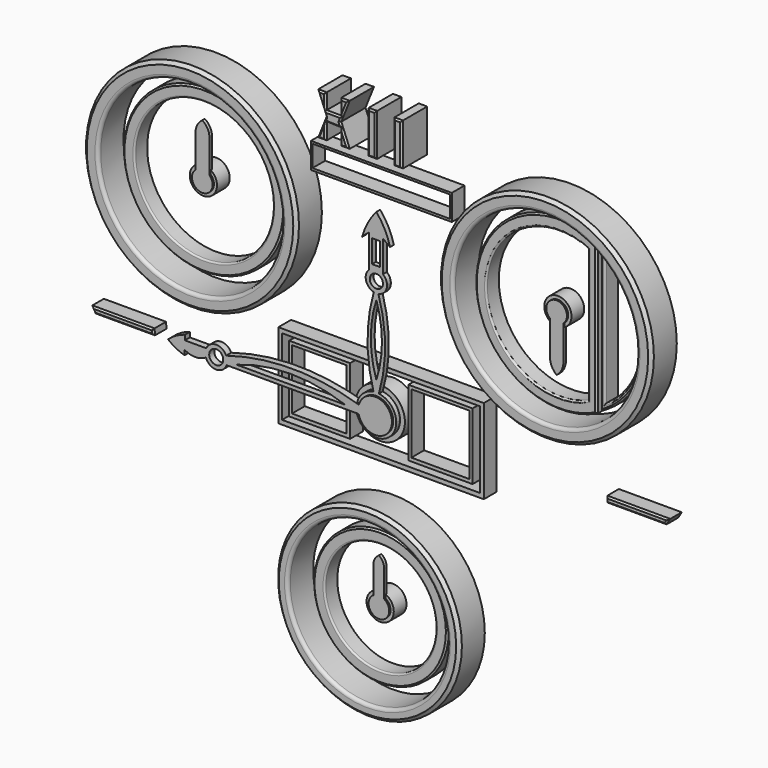
from build123d import *

# Parameters (mm, degrees)
F0_R             = 3.9514377986
F0_R_2           = 2.5863857563
F9_DEPTH         = 2.54
F1_R             = 14.6787999348
F1_R_2           = 12.7425171284
F10_DEPTH        = 5.08
F1_R_3           = 17.0073484495
F1_R_4           = 14.6752720021
F1_R_5           = 17.0023516015
F1_R_6           = 14.6892793779
F1_W             = 1.3462
F1_H             = 6.7620016634
F1_W_2           = 1.3524000533
F2_R             = 2.177276794
F2_R_2           = 1.3961214572
F11_DEPTH        = 2.54
F2_R_3           = 2.1717
F2_R_4           = 1.397
F12_DEPTH        = 2.54
F13_START        = 2.54
F13_DEPTH        = 0.762
F5_R             = 12.9377790339
F5_R_2           = 11.0821270388
F14_DEPTH        = 2.54
F5_R_3           = 10.7502912607
F5_R_4           = 8.8849316167
F15_START        = 2.54
F6_R             = 1.1208583818
F15_DEPTH        = 1.016
F7_W             = 10.2515760809
F7_H             = 10.6458668597
F7_W_2           = 9.2743812129
F7_H_2           = 9.6200094558
F16_DEPTH        = 2.54
F7_W_3           = 9.7352196462
F7_W_4           = 8.6983321235
F7_W_5           = 22.5069178268
F7_H_3           = 4.1028223932
F7_W_6           = 21.9573201612
F7_H_4           = 3.4244768322
F17_START        = 2.286
F17_DEPTH        = 0.508
F18_SIZE         = 0.508
F18_2_SIZE       = 0.508
F18_3_SIZE       = 0.508
F19_R            = 0.508
F19_2_R          = 0.508
F19_3_R          = 0.508
F20_SIZE         = 0.254
F20_2_SIZE       = 0.254
F20_3_SIZE       = 0.254
F20_4_SIZE       = 0.254
F21_R            = 0.254
F21_2_R          = 0.254
F21_3_R          = 0.254
F21_4_R          = 0.254
F22_C1_SIZE      = 0.254
F22_C2_SIZE      = 0.254
F22_C3_SIZE      = 0.254
F22_C4_SIZE      = 0.254
F22_2_C1_SIZE    = 0.254
F22_2_C2_SIZE    = 0.254
F22_2_C3_SIZE    = 0.254
F22_2_C4_SIZE    = 0.254
F22_3_T1_DEPTH   = 2.6588161753
F22_3_T3_DEPTH   = 3.1555706541
F22_3_T5_DEPTH   = 2.3183985613
F22_3_T7_DEPTH   = 2.6588164082
F22_3_T12_DEPTH  = 4.9478647113
F22_3_T17_DEPTH  = 4.9478647113
F22_3_T22_DEPTH  = 3.9716552755
F22_3_T27_DEPTH  = 3.6261524815
F22_3_T33_DEPTH  = 3.8928498877
F22_3_T38_DEPTH  = 4.9478646249
F22_3_T43_DEPTH  = 4.9478646249
F22_3_T49_DEPTH  = 3.1555706541
F22_3_T54_DEPTH  = 2.9716060403
F22_3_T62_DEPTH  = 2.9716060403
F22_3_T67_DEPTH  = 3.1555706541
F22_3_T75_DEPTH  = 4.9478647113
F22_3_T79_DEPTH  = 4.9478647113
F22_3_T86_DEPTH  = 3.3184477965
F22_3_T91_DEPTH  = 3.6261524815
F22_3_T99_DEPTH  = 3.6261524815
F22_3_T104_DEPTH = 3.2396424088
F22_3_T112_DEPTH = 4.9478646249
F22_3_T116_DEPTH = 4.9478646249
F22_4_C1_SIZE    = 0.254
F22_4_C2_SIZE    = 0.254
F22_4_C3_SIZE    = 0.254
F22_4_C4_SIZE    = 0.254
F22_5_C1_SIZE    = 0.254
F22_5_C2_SIZE    = 0.254
F22_5_C3_SIZE    = 0.254
F22_5_C4_SIZE    = 0.254


# Not quite as in the source:
# - a fillet or chamfer that OpenCascade refuses, or shapes differently, is made with other operations: its cross-section is extruded or revolved along the edge and cut away or added


with BuildPart() as f9:
    # F0 (on Front) → F9 (new body)
    with BuildSketch(Plane.XZ):
        Circle(F0_R)
        Circle(F0_R_2, mode=Mode.SUBTRACT)
    extrude(amount=F9_DEPTH)


with BuildPart() as f10:
    # F1 (on Front) → F10 (new body)
    with BuildSketch(Plane.XZ):
        with Locations((0, -27.1976441145)):
            Circle(F1_R)
        with Locations((0, -27.1976441145)):
            Circle(F1_R_2, mode=Mode.SUBTRACT)
    extrude(amount=F10_DEPTH)

    # F18
    f18_edges = [f10.edges().sort_by_distance(p)[0] for p in [
        (-14.6788, -5.08, -27.197644),
    ]]
    chamfer(f18_edges, length=F18_SIZE)

    # F19
    f19_edges = [f10.edges().sort_by_distance(p)[0] for p in [
        (-12.742517, -5.08, -27.197644),
    ]]
    fillet(f19_edges, radius=F19_R)


with BuildPart() as f10b:
    # F1 (on Front) → F10, piece 2 (new body)
    with BuildSketch(Plane.XZ):
        with Locations((-28.3488668501, 23.4561692923)):
            Circle(F1_R_3)
        with Locations((-28.3488668501, 23.4561692923)):
            Circle(F1_R_4, mode=Mode.SUBTRACT)
    extrude(amount=F10_DEPTH)

    # F18#2
    f18_2_edges = [f10b.edges().sort_by_distance(p)[0] for p in [
        (-45.356215, -5.08, 23.456169),
    ]]
    chamfer(f18_2_edges, length=F18_2_SIZE)

    # F19#2
    f19_2_edges = [f10b.edges().sort_by_distance(p)[0] for p in [
        (-43.024139, -5.08, 23.456169),
    ]]
    fillet(f19_2_edges, radius=F19_2_R)


with BuildPart() as f10c:
    # F1 (on Front) → F10, piece 3 (new body)
    with BuildSketch(Plane.XZ):
        with Locations((28.3464, 23.4561692923)):
            Circle(F1_R_5)
        with Locations((28.3464, 23.4561692923)):
            Circle(F1_R_6, mode=Mode.SUBTRACT)
    extrude(amount=F10_DEPTH)

    # F18#3
    f18_3_edges = [f10c.edges().sort_by_distance(p)[0] for p in [
        (11.344048, -5.08, 23.456169),
    ]]
    chamfer(f18_3_edges, length=F18_3_SIZE)

    # F19#3
    f19_3_edges = [f10c.edges().sort_by_distance(p)[0] for p in [
        (13.657121, -5.08, 23.456169),
    ]]
    fillet(f19_3_edges, radius=F19_3_R)


with BuildPart() as f10d:
    # F1 (on Front) → F10, piece 4 (new body)
    with BuildSketch(Plane.XZ):
        with Locations((0.6731, 40.4530894011)):
            Rectangle(F1_W, F1_H)
    extrude(amount=F10_DEPTH)

    # F22: chamfer of 0.254 on 4 edges, made by hand

    # F22_c1
    f22_c1_edges = [f10d.edges().sort_by_distance(p)[0] for p in [
        (0.6731, -5.08, 43.8340902328),
    ]]
    chamfer(f22_c1_edges, length=F22_C1_SIZE)

    # F22_c2
    f22_c2_edges = [f10d.edges().sort_by_distance(p)[0] for p in [
        (0, -5.08, 40.3260894011),
    ]]
    chamfer(f22_c2_edges, length=F22_C2_SIZE)

    # F22_c3
    f22_c3_edges = [f10d.edges().sort_by_distance(p)[0] for p in [
        (0.8001, -5.08, 37.0720885694),
    ]]
    chamfer(f22_c3_edges, length=F22_C3_SIZE)

    # F22_c4
    f22_c4_edges = [f10d.edges().sort_by_distance(p)[0] for p in [
        (1.3462, -5.08, 40.4530894011),
    ]]
    chamfer(f22_c4_edges, length=F22_C4_SIZE)


with BuildPart() as f10e:
    # F1 (on Front) → F10, piece 5 (new body)
    with BuildSketch(Plane.XZ):
        with Locations((4.7994630877, 40.4530894011)):
            Rectangle(F1_W_2, F1_H)
    extrude(amount=F10_DEPTH)

    # F22#2: chamfer of 0.254 on 4 edges, made by hand

    # F22_2_c1
    f22_2_c1_edges = [f10e.edges().sort_by_distance(p)[0] for p in [
        (4.7994630877, -5.08, 43.8340902328),
    ]]
    chamfer(f22_2_c1_edges, length=F22_2_C1_SIZE)

    # F22_2_c2
    f22_2_c2_edges = [f10e.edges().sort_by_distance(p)[0] for p in [
        (4.123263061, -5.08, 40.3260894011),
    ]]
    chamfer(f22_2_c2_edges, length=F22_2_C2_SIZE)

    # F22_2_c3
    f22_2_c3_edges = [f10e.edges().sort_by_distance(p)[0] for p in [
        (4.9264630877, -5.08, 37.0720885694),
    ]]
    chamfer(f22_2_c3_edges, length=F22_2_C3_SIZE)

    # F22_2_c4
    f22_2_c4_edges = [f10e.edges().sort_by_distance(p)[0] for p in [
        (5.4756631143, -5.08, 40.4530894011),
    ]]
    chamfer(f22_2_c4_edges, length=F22_2_C4_SIZE)


with BuildPart() as f10f:
    # F1 (on Front) → F10, piece 6 (new body)
    with BuildSketch(Plane.XZ):
        Polygon((-3.0251389835, 43.8340902328), (-4.3775402009, 43.8340902328), (-4.3775402009, 41.3317270577), (-4.3775402009, 40.4530894011), align=None)
        Polygon((-4.3775402009, 40.4530894011), (-4.3775402009, 41.3317270577), (-6.6959387623, 41.3317270577), (-6.6959387623, 40.4530894011), (-6.6959387623, 39.737328887), (-4.3775402009, 39.6585234992), align=None)
        Polygon((-3.0251389835, 37.0720885694), (-4.3775402009, 40.4530894011), (-4.3775402009, 39.6585234992), (-4.3775402009, 37.0720885694), align=None)
        Polygon((-6.6959387623, 40.4530894011), (-6.6959387623, 41.3317270577), (-6.6959387623, 43.8340902328), (-8.0483402126, 43.8340902328), align=None)
        Polygon((-6.6959387623, 39.737328887), (-6.6959387623, 40.4530894011), (-8.0483402126, 37.0720885694), (-6.6959387623, 37.0720885694), align=None)
    extrude(amount=F10_DEPTH)

    # F22#3: chamfer of 0.254 on 14 edges, made by hand

    # F22_3_s2 → F22_3_t1 (cut)
    with BuildSketch(Plane.YZ.offset(-5.0307476799)):
        Polygon((-4.826, 43.8340902328), (-5.08, 43.5800902328), (-5.08, 43.8340902328), align=None)
        Polygon((-4.826, 37.0720885694), (-5.08, 37.3260885694), (-5.08, 37.0720885694), align=None)
    extrude(amount=F22_3_T1_DEPTH, mode=Mode.SUBTRACT)

    # F22_3_s4 → F22_3_t3 (cut)
    with BuildSketch(Plane.XY.offset(41.3317270577)):
        Polygon((-4.3775402009, -4.826), (-4.1235402009, -5.08), (-4.3775402009, -5.08), align=None)
        Polygon((-6.6959387623, -4.826), (-6.9499387623, -5.08), (-6.6959387623, -5.08), align=None)
    extrude(amount=F22_3_T3_DEPTH, mode=Mode.SUBTRACT)

    # F22_3_s6 → F22_3_t5 (cut)
    with BuildSketch(Plane.YZ.offset(-6.6959387623)):
        Polygon((-4.826, 41.3317270577), (-5.08, 41.0777270577), (-5.08, 41.3317270577), align=None)
    extrude(amount=F22_3_T5_DEPTH, mode=Mode.SUBTRACT)

    # F22_3_s8 → F22_3_t7 (cut)
    with BuildSketch(Plane.YZ.offset(-8.7015476915)):
        Polygon((-4.826, 43.8340902328), (-5.08, 43.5800902328), (-5.08, 43.8340902328), align=None)
        Polygon((-4.826, 37.0720885694), (-5.08, 37.3260885694), (-5.08, 37.0720885694), align=None)
    extrude(amount=F22_3_T7_DEPTH, mode=Mode.SUBTRACT)


with BuildPart() as f11:
    # F2 (on Front) → F11 (new body)
    with BuildSketch(Plane.XZ):
        with Locations((-28.2395668328, 23.5069990158)):
            Circle(F2_R)
        with Locations((-28.2395668328, 23.5069990158)):
            Circle(F2_R_2, mode=Mode.SUBTRACT)
    extrude(amount=F11_DEPTH)


with BuildPart() as f11b:
    # F2 (on Front) → F11, piece 2 (new body)
    with BuildSketch(Plane.XZ):
        with Locations((28.380965814, 23.5069990158)):
            Circle(F2_R)
        with Locations((28.380965814, 23.5069990158)):
            Circle(F2_R_2, mode=Mode.SUBTRACT)
    extrude(amount=F11_DEPTH)


with BuildPart() as f11c:
    # F2 (on Front) → F11, piece 3 (new body)
    with BuildSketch(Plane.XZ):
        with Locations((0, -27.2187907249)):
            Circle(F2_R_3)
        with Locations((0, -27.2187907249)):
            Circle(F2_R_4, mode=Mode.SUBTRACT)
    extrude(amount=F11_DEPTH)


with BuildPart() as f11d:
    # F2 (on Front) → F11, piece 4 (new body)
    with BuildSketch(Plane.XZ):
        Polygon((-46.1701489985, 0), (-45.6411466002, -0.9652937879), (-36.1669466002, -0.9652937879), (-36.2358952414, 0), align=None)
    extrude(amount=F11_DEPTH)

    # F22#4: chamfer of 0.254 on 4 edges, made by hand

    # F22_4_c1
    f22_4_c1_edges = [f11d.edges().sort_by_distance(p)[0] for p in [
        (-36.2014209208, -2.54, -0.4826468939),
    ]]
    chamfer(f22_4_c1_edges, length=F22_4_C1_SIZE)

    # F22_4_c2
    f22_4_c2_edges = [f11d.edges().sort_by_distance(p)[0] for p in [
        (-41.3303456788, -2.54, 0),
    ]]
    chamfer(f22_4_c2_edges, length=F22_4_C2_SIZE)

    # F22_4_c3
    f22_4_c3_edges = [f11d.edges().sort_by_distance(p)[0] for p in [
        (-45.8360489835, -2.54, -0.6096468939),
    ]]
    chamfer(f22_4_c3_edges, length=F22_4_C3_SIZE)

    # F22_4_c4
    f22_4_c4_edges = [f11d.edges().sort_by_distance(p)[0] for p in [
        (-40.8865495971, -2.54, -0.9652937879),
    ]]
    chamfer(f22_4_c4_edges, length=F22_4_C4_SIZE)


with BuildPart() as f11e:
    # F2 (on Front) → F11, piece 5 (new body)
    with BuildSketch(Plane.XZ):
        Polygon((36.0910706222, -0.9652937879), (45.5532521009, -0.9652937879), (46.1384877563, 0), (36.0910706222, 0), align=None)
    extrude(amount=F11_DEPTH)

    # F22#5: chamfer of 0.254 on 4 edges, made by hand

    # F22_5_c1
    f22_5_c1_edges = [f11e.edges().sort_by_distance(p)[0] for p in [
        (45.8458699286, -2.54, -0.4826468939),
    ]]
    chamfer(f22_5_c1_edges, length=F22_5_C1_SIZE)

    # F22_5_c2
    f22_5_c2_edges = [f11e.edges().sort_by_distance(p)[0] for p in [
        (40.9662612768, -2.54, 0),
    ]]
    chamfer(f22_5_c2_edges, length=F22_5_C2_SIZE)

    # F22_5_c3
    f22_5_c3_edges = [f11e.edges().sort_by_distance(p)[0] for p in [
        (36.0910706222, -2.54, -0.6096468939),
    ]]
    chamfer(f22_5_c3_edges, length=F22_5_C3_SIZE)

    # F22_5_c4
    f22_5_c4_edges = [f11e.edges().sort_by_distance(p)[0] for p in [
        (40.8006434492, -2.54, -0.9652937879),
    ]]
    chamfer(f22_5_c4_edges, length=F22_5_C4_SIZE)


with BuildPart() as f12:
    # F3 (on Front) → F12 (new body)
    with BuildSketch(Plane.XZ):
        Polygon((-16.2610244006, 6.7634354346), (-16.2610244006, 0), (-15.6719069928, 0), (-15.6719069928, 6.1107245274), (15.9075018018, 6.1107245274), (15.9075018018, 0), (16.5488310158, 0), (16.5488310158, 6.7634354346), align=None)
        Polygon((-15.6719069928, 0), (-16.2610244006, 0), (-16.2610244006, -6.7634354346), (16.5488310158, -6.7634354346), (16.5488310158, 0), (15.9075018018, 0), (15.9075018018, -6.0778195038), (-15.6719069928, -6.0778195038), align=None)
    extrude(amount=F12_DEPTH)


with BuildPart() as f12b:
    # F3 (on Front) → F12, piece 2 (new body)
    with BuildSketch(Plane.XZ):
        with BuildLine():
            ThreePointArc((35.9539873898, 34.7763706712), (35.5764961596, 34.9957570446), (35.1919867098, 35.2025963366))
            Line((35.1919867098, 35.2025963366), (35.1919867098, 34.3377191043))
            Line((35.1919867098, 34.3377191043), (35.1919867098, 12.5088718319))
            Line((35.1919867098, 12.5088718319), (35.1919867098, 11.6439945996))
            ThreePointArc((35.1919867098, 11.6439945996), (35.5764961596, 11.8508338916), (35.9539873898, 12.070220265))
            ThreePointArc((35.9539873898, 12.070220265), (42.3632363542, 23.4232954681), (35.9539873898, 34.7763706712))
        make_face()
        with BuildLine():
            ThreePointArc((35.9539873898, 33.8762869503), (41.6012369096, 23.4232954681), (35.9539873898, 12.9703039859))
            Line((35.9539873898, 12.9703039859), (35.9539873898, 33.8762869503))
        make_face(mode=Mode.SUBTRACT)
    extrude(amount=F12_DEPTH)

    # F20
    f20_edges = [f12b.edges().sort_by_distance(p)[0] for p in [
        (42.363236, -2.54, 23.423295),
        (35.191987, -2.54, 23.423295),
    ]]
    chamfer(f20_edges, length=F20_SIZE)

    # F21
    f21_edges = [f12b.edges().sort_by_distance(p)[0] for p in [
        (41.601237, -2.54, 23.423295),
        (35.953987, -2.54, 23.423295),
    ]]
    fillet(f21_edges, radius=F21_R)


with BuildPart() as f13:
    # F4 (on Front) → F13 (new body)
    with BuildSketch(Plane.XZ.offset(F13_START)):
        with BuildLine():
            ThreePointArc((-0.4558769655, 3.1394309196), (-2.0757704263, -2.3989638271), (3.1723572161, 0))
            ThreePointArc((3.1723572161, 0), (2.3824784995, 2.0946709779), (0.406182913, 3.1462462948))
            ThreePointArc((0.406182913, 3.1462462948), (0.2035106502, 3.1658227559), (0, 3.1723572161))
            ThreePointArc((0, 3.1723572161), (-0.2285322453, 3.1641149346), (-0.4558769655, 3.1394309196))
        make_face()
        with BuildLine():
            ThreePointArc((0, 3.1723572161), (0.2035106502, 3.1658227559), (0.406182913, 3.1462462948))
            ThreePointArc((0.406182913, 3.1462462948), (1.391187797, 10.149801888), (0.3357800332, 17.1430943901))
            ThreePointArc((0.3357800332, 17.1430943901), (0.1687169951, 17.118088395), (0, 17.1097257365))
            Line((0, 17.1097257365), (0, 16.1932520568))
            ThreePointArc((0, 16.1932520568), (0.8887872407, 10.5615877546), (0, 4.9299234524))
            Line((0, 4.9299234524), (0, 3.1723572161))
        make_face()
        with BuildLine():
            ThreePointArc((-0.4104431947, 17.1598319675), (-1.4162135324, 10.1528170746), (-0.4558769655, 3.1394309196))
            ThreePointArc((-0.4558769655, 3.1394309196), (-0.2285322453, 3.1641149346), (0, 3.1723572161))
            Line((0, 3.1723572161), (0, 4.9299234524))
            ThreePointArc((0, 4.9299234524), (-0.8887097505, 10.5615877546), (0, 16.1932520568))
            Line((0, 16.1932520568), (0, 17.1097257365))
            ThreePointArc((0, 17.1097257365), (-0.2067451635, 17.1222986209), (-0.4104431947, 17.1598319675))
        make_face()
        with BuildLine():
            ThreePointArc((0, 17.1097257365), (0.1687169951, 17.118088395), (0.3357800332, 17.1430943901))
            ThreePointArc((0.3357800332, 17.1430943901), (0.5986404515, 17.2181991689), (0.8461306577, 17.3343237793))
            ThreePointArc((0.8461306577, 17.3343237793), (0.9616142265, 17.4065401841), (1.0709691316, 17.4877385125))
            ThreePointArc((1.0709691316, 17.4877385125), (1.5391615871, 18.0797597987), (1.7061176519, 18.8158433884))
            ThreePointArc((1.7061176519, 18.8158433884), (1.5351225156, 19.5603138744), (1.0564129803, 20.1555556924))
            ThreePointArc((1.0564129803, 20.1555556924), (0.5590754117, 20.4277590581), (0, 20.5219610404))
            Line((0, 20.5219610404), (0, 19.8668396389))
            ThreePointArc((0, 19.8668396389), (0.7431665757, 19.5590099641), (1.0509962505, 18.8158433884))
            ThreePointArc((1.0509962505, 18.8158433884), (0.7431665757, 18.0726768127), (0, 17.764847138))
            Line((0, 17.764847138), (0, 17.1097257365))
        make_face()
        with BuildLine():
            ThreePointArc((-0.980104729, 17.419336259), (-0.7072775278, 17.263233991), (-0.4104431947, 17.1598319675))
            ThreePointArc((-0.4104431947, 17.1598319675), (-0.2067451635, 17.1222986209), (0, 17.1097257365))
            Line((0, 17.1097257365), (0, 17.764847138))
            ThreePointArc((0, 17.764847138), (-1.0509962505, 18.8158433884), (0, 19.8668396389))
            Line((0, 19.8668396389), (0, 20.5219610404))
            ThreePointArc((0, 20.5219610404), (-0.6555211315, 20.3910035354), (-1.2104097987, 20.0182349892))
            ThreePointArc((-1.2104097987, 20.0182349892), (-1.6994578919, 18.6652435349), (-0.980104729, 17.419336259))
        make_face()
        with BuildLine():
            Line((-1.2104097987, 25.1528434455), (-1.2104097987, 20.0182349892))
            ThreePointArc((-1.2104097987, 20.0182349892), (-0.6555211315, 20.3910035354), (0, 20.5219610404))
            Line((0, 20.5219610404), (0, 21.0046619177))
            Line((0, 21.0046619177), (-0.6953111151, 21.0046619177))
            Line((-0.6953111151, 21.0046619177), (-0.6953111151, 24.6570892632))
            Line((-0.6953111151, 24.6570892632), (0, 24.6570892632))
            Line((0, 24.6570892632), (0, 25.8310846984))
            ThreePointArc((0, 25.8310846984), (-0.6248635953, 25.5854711733), (-1.2104097987, 25.2569652219))
            Line((-1.2104097987, 25.2569652219), (-1.2104097987, 25.1528434455))
        make_face()
        with BuildLine():
            Line((0, 21.0046619177), (0, 20.5219610404))
            ThreePointArc((0, 20.5219610404), (0.5590754117, 20.4277590581), (1.0564129803, 20.1555556924))
            Line((1.0564129803, 20.1555556924), (1.0564129803, 25.1528434455))
            ThreePointArc((1.0564129803, 25.1528434455), (0.5332923964, 25.4998857627), (0, 25.8310846984))
            Line((0, 25.8310846984), (0, 24.6570892632))
            Line((0, 24.6570892632), (0.5439050728, 24.6570892632))
            Line((0.5439050728, 24.6570892632), (0.5439050728, 21.0046619177))
            Line((0.5439050728, 21.0046619177), (0, 21.0046619177))
        make_face()
        with BuildLine():
            ThreePointArc((-2.2606367711, 24.3309792131), (-1.768676428, 24.8315735687), (-1.2104097987, 25.2569652219))
            ThreePointArc((-1.2104097987, 25.2569652219), (-0.6248635953, 25.5854711733), (0, 25.8310846984))
            ThreePointArc((0, 25.8310846984), (0.5332923964, 25.4998857627), (1.0564129803, 25.1528434455))
            ThreePointArc((1.0564129803, 25.1528434455), (1.6222464053, 24.7511786169), (2.1744552068, 24.3309792131))
            ThreePointArc((2.1744552068, 24.3309792131), (1.3353719943, 26.5779681689), (0, 28.5704042763))
            ThreePointArc((0, 28.5704042763), (-1.3834310278, 26.5856618734), (-2.2606367711, 24.3309792131))
        make_face()
    extrude(amount=F13_DEPTH)


with BuildPart() as f14:
    # F5 (on Front) → F14 (new body)
    with BuildSketch(Plane.XZ):
        with Locations((-28.175085783, 23.5215127468)):
            Circle(F5_R)
        with Locations((-28.175085783, 23.5215127468)):
            Circle(F5_R_2, mode=Mode.SUBTRACT)
    extrude(amount=F14_DEPTH)

    # F20#2
    f20_2_edges = [f14.edges().sort_by_distance(p)[0] for p in [
        (-41.112865, -2.54, 23.521513),
    ]]
    chamfer(f20_2_edges, length=F20_2_SIZE)

    # F21#2
    f21_2_edges = [f14.edges().sort_by_distance(p)[0] for p in [
        (-39.257213, -2.54, 23.521513),
    ]]
    fillet(f21_2_edges, radius=F21_2_R)


with BuildPart() as f14b:
    # F5 (on Front) → F14, piece 2 (new body)
    with BuildSketch(Plane.XZ):
        with Locations((0, -27.3638349026)):
            Circle(F5_R_3)
        with Locations((0, -27.3638349026)):
            Circle(F5_R_4, mode=Mode.SUBTRACT)
    extrude(amount=F14_DEPTH)

    # F20#3
    f20_3_edges = [f14b.edges().sort_by_distance(p)[0] for p in [
        (-10.750291, -2.54, -27.363835),
    ]]
    chamfer(f20_3_edges, length=F20_3_SIZE)

    # F21#3
    f21_3_edges = [f14b.edges().sort_by_distance(p)[0] for p in [
        (-8.884932, -2.54, -27.363835),
    ]]
    fillet(f21_3_edges, radius=F21_3_R)


with BuildPart() as f14c:
    # F5 (on Front) → F14, piece 3 (new body)
    with BuildSketch(Plane.XZ):
        with BuildLine():
            Line((34.5556773245, 11.0531123355), (34.5556773245, 35.4083329439))
            ThreePointArc((34.5556773245, 35.4083329439), (15.1532113023, 23.2307226397), (34.5556773245, 11.0531123355))
        make_face()
        with BuildLine():
            ThreePointArc((33.233191818, 12.5319492072), (16.9140992275, 23.1922352687), (33.233191818, 33.8525213301))
            Line((33.233191818, 33.8525213301), (33.233191818, 12.5319492072))
        make_face(mode=Mode.SUBTRACT)
    extrude(amount=F14_DEPTH)

    # F20#4
    f20_4_edges = [f14c.edges().sort_by_distance(p)[0] for p in [
        (15.153211, -2.54, 23.230723),
        (34.555677, -2.54, 23.230723),
    ]]
    chamfer(f20_4_edges, length=F20_4_SIZE)

    # F21#4
    f21_4_edges = [f14c.edges().sort_by_distance(p)[0] for p in [
        (16.914099, -2.54, 23.192235),
        (33.233192, -2.54, 23.192235),
    ]]
    fillet(f21_4_edges, radius=F21_4_R)


with BuildPart() as f15:
    # F6 (on Front) → F15 (new body)
    with BuildSketch(Plane.XZ.offset(F15_START)):
        with BuildLine():
            ThreePointArc((-2.5908380434, 0.7330955651), (-2.6670070938, 0.3700595032), (-2.6925584254, 0))
            ThreePointArc((-2.6925584254, 0), (-2.6762037781, -0.2963177559), (-2.6273385129, -0.5890358333))
            ThreePointArc((-2.6273385129, -0.5890358333), (0.2963177559, -2.6762037781), (2.6925584254, 0))
            ThreePointArc((2.6925584254, 0), (0.3700595032, 2.6670070938), (-2.5908380434, 0.7330955651))
        make_face()
        with BuildLine():
            Line((-4.7591174953, 0), (-2.6925584254, 0))
            ThreePointArc((-2.6925584254, 0), (-2.6670070938, 0.3700595032), (-2.5908380434, 0.7330955651))
            Line((-2.5908380434, 0.7330955651), (-2.6273385129, 0.7338119022))
            ThreePointArc((-2.6273385129, 0.7338119022), (-13.2059349065, 2.3258538257), (-23.7845313001, 0.7338119022))
            ThreePointArc((-23.7845313001, 0.7338119022), (-23.6641674264, 0.375645672), (-23.6234140265, 0))
            Line((-23.6234140265, 0), (-22.1354551613, 0))
            ThreePointArc((-22.1354551613, 0), (-13.4472863283, 1.5235018353), (-4.7591174953, 0))
        make_face()
        with BuildLine():
            ThreePointArc((-2.6273385129, -0.5890358333), (-2.6762037781, -0.2963177559), (-2.6925584254, 0))
            Line((-2.6925584254, 0), (-4.7591174953, 0))
            Line((-4.7591174953, 0), (-22.1354551613, 0))
            Line((-22.1354551613, 0), (-23.6234140265, 0))
            ThreePointArc((-23.6234140265, 0), (-23.6491049134, -0.2989018406), (-23.7254239693, -0.5890358333))
            Line((-23.7254239693, -0.5890358333), (-2.6273385129, -0.5890358333))
        make_face()
        with BuildLine():
            ThreePointArc((-27.0246826038, -0.5890358333), (-25.3750532866, -1.75163926), (-23.7254239693, -0.5890358333))
            ThreePointArc((-23.7254239693, -0.5890358333), (-23.6491049134, -0.2989018406), (-23.6234140265, 0))
            ThreePointArc((-23.6234140265, 0), (-23.6641674264, 0.375645672), (-23.7845313001, 0.7338119022))
            ThreePointArc((-23.7845313001, 0.7338119022), (-25.3750532866, 1.75163926), (-26.965575273, 0.7338119022))
            ThreePointArc((-26.965575273, 0.7338119022), (-27.0856877882, 0.3767886662), (-27.1266909828, 0.0023406119))
            ThreePointArc((-27.1266909828, 0.0023406119), (-27.101200977, -0.2977486323), (-27.0246826038, -0.5890358333))
        make_face()
        with Locations((-25.3750532866, 0)):
            Circle(F6_R, mode=Mode.SUBTRACT)
        with BuildLine():
            ThreePointArc((-30.4154170935, -0.5986585686), (-28.7186605171, -1.0834018075), (-27.0246826038, -0.5890358333))
            ThreePointArc((-27.0246826038, -0.5890358333), (-27.101200977, -0.2977486323), (-27.1266909828, 0.0023406119))
            Line((-27.1266909828, 0.0023406119), (-30.4021472575, 0.0774969087))
            Line((-30.4021472575, 0.0774969087), (-30.4154170935, -0.5986585686))
        make_face()
        with BuildLine():
            Line((-30.4021472575, 0.0774969087), (-27.1266909828, 0.0023406119))
            ThreePointArc((-27.1266909828, 0.0023406119), (-27.0856877882, 0.3767886662), (-26.965575273, 0.7338119022))
            Line((-26.965575273, 0.7338119022), (-30.3892667994, 0.7338119022))
            Line((-30.3892667994, 0.7338119022), (-30.4021472575, 0.0774969087))
        make_face()
        with BuildLine():
            Line((-30.4306899177, -1.3768749559), (-30.4154170935, -0.5986585686))
            Line((-30.4154170935, -0.5986585686), (-30.4021472575, 0.0774969087))
            Line((-30.4021472575, 0.0774969087), (-30.3892667994, 0.7338119022))
            Line((-30.3892667994, 0.7338119022), (-30.3735788912, 1.5331786126))
            ThreePointArc((-30.3735788912, 1.5331786126), (-31.8083059454, 0.9188007355), (-33.069934696, 0))
            ThreePointArc((-33.069934696, 0), (-31.8247897317, -0.8311985571), (-30.4306899177, -1.3768749559))
        make_face()
    extrude(amount=F15_DEPTH)

    # F7 (on Front) → F16, piece 2 (join)
    with BuildSketch(Plane.XZ):
        with Locations((-9.674514411, 0.1040718053)):
            Rectangle(F7_W_3, F7_H)
        with Locations((-9.7321192734, 0.1409782562)):
            Rectangle(F7_W_4, F7_H_2, mode=Mode.SUBTRACT)
    extrude(amount=F16_DEPTH)


with BuildPart() as f16:
    # F7 (on Front) → F16 (new body)
    with BuildSketch(Plane.XZ):
        with Locations((9.6296481788, 0.1040718053)):
            Rectangle(F7_W, F7_H)
        with Locations((9.6231098287, 0.1409782562)):
            Rectangle(F7_W_2, F7_H_2, mode=Mode.SUBTRACT)
    extrude(amount=F16_DEPTH)


with BuildPart() as f16b:
    # F7 (on Front) → F16, piece 3 (new body)
    with BuildSketch(Plane.XZ):
        with Locations((0.1843241043, 32.6070804149)):
            Rectangle(F7_W_5, F7_H_3)
        with Locations((0.1655607484, 32.6248798519)):
            Rectangle(F7_W_6, F7_H_4, mode=Mode.SUBTRACT)
    extrude(amount=F16_DEPTH)


with BuildPart() as f17:
    # F8 (on Front) → F17 (new body)
    with BuildSketch(Plane.XZ.offset(F17_START)):
        with BuildLine():
            ThreePointArc((-0.887707951, -25.8237374084), (-0.7942761489, -28.6646606978), (1.6516435072, -27.2165406495))
            ThreePointArc((1.6516435072, -27.2165406495), (1.43558942, -26.3998342811), (0.8439519087, -25.7967972041))
            ThreePointArc((0.8439519087, -25.7967972041), (-0.0256922452, -25.5650969831), (-0.887707951, -25.8237374084))
        make_face()
        with BuildLine():
            ThreePointArc((-0.887707951, -25.8237374084), (-0.0256922452, -25.5650969831), (0.8439519087, -25.7967972041))
            Line((0.8439519087, -25.7967972041), (0.8439519087, -21.5243733251))
            ThreePointArc((0.8439519087, -21.5243733251), (0.6197614501, -20.628145968), (0, -19.9430324137))
            ThreePointArc((0, -19.9430324137), (-0.6506062746, -20.6176395598), (-0.887707951, -21.5243733251))
            Line((-0.887707951, -21.5243733251), (-0.887707951, -25.8237374084))
        make_face()
    extrude(amount=F17_DEPTH)


with BuildPart() as f17b:
    # F8 (on Front) → F17, piece 2 (new body)
    with BuildSketch(Plane.XZ.offset(F17_START)):
        with BuildLine():
            ThreePointArc((-29.2991695786, 24.7656393852), (-28.8883739633, 22.0251706743), (-26.5601845461, 23.5279866413))
            ThreePointArc((-26.5601845461, 23.5279866413), (-26.6911895921, 24.1721321539), (-27.063390799, 24.7139365698))
            ThreePointArc((-27.063390799, 24.7139365698), (-28.1711773316, 25.1766646469), (-29.2991695786, 24.7656393852))
        make_face()
        with BuildLine():
            ThreePointArc((-29.2991695786, 24.7656393852), (-28.1711773316, 25.1766646469), (-27.063390799, 24.7139365698))
            Line((-27.063390799, 24.7139365698), (-27.063390799, 29.9920143188))
            ThreePointArc((-27.063390799, 29.9920143188), (-27.3687232231, 31.1821967987), (-28.2093033284, 32.0784039795))
            ThreePointArc((-28.2093033284, 32.0784039795), (-29.0102881388, 31.168962731), (-29.2991695786, 29.9920143188))
            Line((-29.2991695786, 29.9920143188), (-29.2991695786, 24.7656393852))
        make_face()
    extrude(amount=F17_DEPTH)


with BuildPart() as f17c:
    # F8 (on Front) → F17, piece 3 (new body)
    with BuildSketch(Plane.XZ.offset(F17_START)):
        with BuildLine():
            ThreePointArc((29.4718204175, 22.2740400105), (29.887661451, 22.8334801104), (30.0350634186, 23.5147800814))
            ThreePointArc((30.0350634186, 23.5147800814), (27.6889425323, 25.0079270572), (27.3297089223, 22.2502609573))
            ThreePointArc((27.3297089223, 22.2502609573), (28.4051547156, 21.8666777414), (29.4718204175, 22.2740400105))
        make_face()
        with BuildLine():
            ThreePointArc((29.4718204175, 22.2740400105), (28.4051547156, 21.8666777414), (27.3297089223, 22.2502609573))
            Line((27.3297089223, 22.2502609573), (27.3297089223, 16.8453882873))
            ThreePointArc((27.3297089223, 16.8453882873), (27.607744525, 15.6263428574), (28.3868595367, 14.648408629))
            ThreePointArc((28.3868595367, 14.648408629), (29.1857963033, 15.620249547), (29.4718204175, 16.8453882873))
            Line((29.4718204175, 16.8453882873), (29.4718204175, 22.2740400105))
        make_face()
    extrude(amount=F17_DEPTH)


with BuildPart() as f22_3_tool10:
    # F22_3_s11 → F22_3_t12 (new body)
    with BuildSketch(Plane(origin=(-16.4679253869, 0, 41.1697794457), x_dir=(0, 1, 0), z_dir=(0.3713909409, 0, -0.9284765851))):
        Polygon((-4.826, 8.8068885804), (-5.08, 9.0608885804), (-5.08, 8.8068885804), align=None)
    extrude(amount=F22_3_T12_DEPTH)

    split(bisect_by=Plane(origin=(-19.7217092063, 0, 7.8886902015), x_dir=(0, 1, 0), z_dir=(-0.9284765851, 0, 0.3713909409)), keep=Keep.TOP)


with BuildPart() as f10f_1:
    add(f10f.part)

    # F22_3_t9: cut F22_3_tool10
    add(f22_3_tool10.part, mode=Mode.SUBTRACT)


with BuildPart() as f22_3_tool15:
    # F22_3_s16 → F22_3_t17 (new body)
    with BuildSketch(Plane(origin=(13.2683657842, 0, 33.170887049), x_dir=(0, 1, 0), z_dir=(-0.3713909409, 0, -0.9284765851))):
        Polygon((-4.826, -21.2409332919), (-5.08, -20.9869332919), (-5.08, -21.2409332919), align=None)
    extrude(amount=F22_3_T17_DEPTH)

    split(bisect_by=Plane(origin=(8.1769898341, 0, 3.2707986365), x_dir=(0, 1, 0), z_dir=(-0.9284765851, 0, -0.3713909409)), keep=Keep.TOP)


with BuildPart() as f10f_2:
    add(f10f_1.part)

    # F22_3_t14: cut F22_3_tool15
    add(f22_3_tool15.part, mode=Mode.SUBTRACT)


with BuildPart() as f22_3_tool20:
    # F22_3_s21 → F22_3_t22 (new body)
    with BuildSketch(Plane.XY.offset(36.4188810905)):
        Polygon((-6.6959387623, -4.826), (-6.9499387623, -5.08), (-6.6959387623, -5.08), align=None)
    extrude(amount=F22_3_T22_DEPTH)

    split(bisect_by=Plane(origin=(1.341437129, 0, 39.4641280085), x_dir=(0, 1, 0), z_dir=(-0.033971683, 0, -0.9994227958)), keep=Keep.TOP)


with BuildPart() as f10f_3:
    add(f10f_2.part)

    # F22_3_t19: cut F22_3_tool20
    add(f22_3_tool20.part, mode=Mode.SUBTRACT)


with BuildPart() as f22_3_tool25:
    # F22_3_s26 → F22_3_t27 (new body)
    with BuildSketch(Plane(origin=(-8.6902063361, 0, 0.2953914359), x_dir=(0, 1, 0), z_dir=(0.9994227958, 0, -0.033971683))):
        Polygon((-4.826, 39.4869200248), (-5.08, 39.7409200248), (-5.08, 39.4869200248), align=None)
    extrude(amount=F22_3_T27_DEPTH)

    split(bisect_by=Plane.YZ.offset(-6.6959387623), keep=Keep.TOP)

    split(bisect_by=Plane.YZ.offset(-4.3775402009), keep=Keep.BOTTOM)


with BuildPart() as f10f_4:
    add(f10f_3.part)

    # F22_3_t24: cut F22_3_tool25
    add(f22_3_tool25.part, mode=Mode.SUBTRACT)


with BuildPart() as f22_3_tool31:
    # F22_3_s32 → F22_3_t33 (new body)
    with BuildSketch(Plane.XY.offset(40.3117309782)):
        Polygon((-4.3775402009, -4.826), (-4.1235402009, -5.08), (-4.3775402009, -5.08), align=None)
    extrude(amount=-F22_3_T33_DEPTH)

    split(bisect_by=Plane(origin=(1.341437129, 0, 39.4641280085), x_dir=(0, 1, 0), z_dir=(-0.033971683, 0, -0.9994227958)), keep=Keep.TOP)


with BuildPart() as f10f_5:
    add(f10f_4.part)

    # F22_3_t30: cut F22_3_tool31
    add(f22_3_tool31.part, mode=Mode.SUBTRACT)


with BuildPart() as f22_3_tool36:
    # F22_3_s37 → F22_3_t38 (new body)
    with BuildSketch(Plane(origin=(-12.958150589, 0, 32.3953552789), x_dir=(0, 1, 0), z_dir=(-0.3713908858, 0, 0.9284766071))):
        Polygon((-4.826, -10.9594650332), (-5.08, -10.7054650332), (-5.08, -10.9594650332), align=None)
    extrude(amount=F22_3_T38_DEPTH)

    split(bisect_by=Plane(origin=(-17.7230886526, 0, 7.0892400989), x_dir=(0, 1, 0), z_dir=(0.9284766071, 0, -0.3713908858)), keep=Keep.TOP)


with BuildPart() as f10f_6:
    add(f10f_5.part)

    # F22_3_t35: cut F22_3_tool36
    add(f22_3_tool36.part, mode=Mode.SUBTRACT)


with BuildPart() as f22_3_tool41:
    # F22_3_s42 → F22_3_t43 (new body)
    with BuildSketch(Plane(origin=(13.1029531475, 0, 32.7573614384), x_dir=(0, 1, 0), z_dir=(0.3713908858, 0, 0.9284766071))):
        Polygon((-4.826, 19.0883523796), (-5.08, 19.3423523796), (-5.08, 19.0883523796), align=None)
    extrude(amount=F22_3_T43_DEPTH)

    split(bisect_by=Plane(origin=(10.1756069097, 0, 4.0702454267), x_dir=(0, 1, 0), z_dir=(0.9284766071, 0, 0.3713908858)), keep=Keep.TOP)


with BuildPart() as f10f_7:
    add(f10f_6.part)

    # F22_3_t40: cut F22_3_tool41
    add(f22_3_tool41.part, mode=Mode.SUBTRACT)


with BuildPart() as f22_3_tool47:
    # F22_3_s48 → F22_3_t49 (new body)
    with BuildSketch(Plane.XY.offset(43.8340902328)):
        Polygon((-4.3775402009, -4.826), (-4.1235402009, -5.08), (-4.3775402009, -5.08), align=None)
    extrude(amount=-F22_3_T49_DEPTH)

    split(bisect_by=Plane.XY.offset(41.3317270577), keep=Keep.BOTTOM)

    split(bisect_by=Plane(origin=(-17.7230886526, 0, 7.0892400989), x_dir=(0, 1, 0), z_dir=(-0.9284766071, 0, 0.3713908858)), keep=Keep.TOP)


with BuildPart() as f22_3_tool52:
    # F22_3_s53 → F22_3_t54 (new body)
    with BuildSketch(Plane.YZ.offset(-3.724332722)):
        Polygon((-4.826, 41.3317270577), (-5.08, 41.0777270577), (-5.08, 41.3317270577), align=None)
    extrude(amount=-F22_3_T54_DEPTH)

    split(bisect_by=Plane.YZ.offset(-4.3775402009), keep=Keep.TOP)

    split(bisect_by=Plane(origin=(-17.7230886526, 0, 7.0892400989), x_dir=(0, 1, 0), z_dir=(-0.9284766071, 0, 0.3713908858)), keep=Keep.TOP)


with BuildPart() as f22_3_tool47_1:
    add(f22_3_tool47.part)

    # F22_3_t57: intersect F22_3_tool52
    add(f22_3_tool52.part, mode=Mode.INTERSECT)


with BuildPart() as f10f_8:
    add(f10f_7.part)

    # F22_3_t45: cut F22_3_tool47
    add(f22_3_tool47_1.part, mode=Mode.SUBTRACT)


with BuildPart() as f22_3_tool60:
    # F22_3_s61 → F22_3_t62 (new body)
    with BuildSketch(Plane.YZ.offset(-4.3775402009)):
        Polygon((-4.826, 41.3317270577), (-5.08, 41.0777270577), (-5.08, 41.3317270577), align=None)
    extrude(amount=-F22_3_T62_DEPTH)

    split(bisect_by=Plane.YZ.offset(-6.6959387623), keep=Keep.BOTTOM)

    split(bisect_by=Plane(origin=(8.1769898341, 0, 3.2707986365), x_dir=(0, 1, 0), z_dir=(0.9284765851, 0, 0.3713909409)), keep=Keep.TOP)


with BuildPart() as f22_3_tool65:
    # F22_3_s66 → F22_3_t67 (new body)
    with BuildSketch(Plane.XY.offset(40.6785195788)):
        Polygon((-6.6959387623, -4.826), (-6.9499387623, -5.08), (-6.6959387623, -5.08), align=None)
    extrude(amount=F22_3_T67_DEPTH)

    split(bisect_by=Plane.XY.offset(41.3317270577), keep=Keep.BOTTOM)

    split(bisect_by=Plane(origin=(8.1769898341, 0, 3.2707986365), x_dir=(0, 1, 0), z_dir=(0.9284765851, 0, 0.3713909409)), keep=Keep.TOP)


with BuildPart() as f22_3_tool60_1:
    add(f22_3_tool60.part)

    # F22_3_t70: intersect F22_3_tool65
    add(f22_3_tool65.part, mode=Mode.INTERSECT)


with BuildPart() as f10f_9:
    add(f10f_8.part)

    # F22_3_t58: cut F22_3_tool60
    add(f22_3_tool60_1.part, mode=Mode.SUBTRACT)


with BuildPart() as f22_3_tool73:
    # F22_3_s74 → F22_3_t75 (new body)
    with BuildSketch(Plane(origin=(-16.4679253869, 0, 41.1697794457), x_dir=(0, 1, 0), z_dir=(0.3713909409, 0, -0.9284765851))):
        Polygon((-4.826, 8.8068885804), (-5.08, 9.0608885804), (-5.08, 8.8068885804), align=None)
    extrude(amount=F22_3_T75_DEPTH)

    split(bisect_by=Plane(origin=(-19.7217092063, 0, 7.8886902015), x_dir=(0, 1, 0), z_dir=(0.9284765851, 0, -0.3713909409)), keep=Keep.TOP)


with BuildPart() as f22_3_tool77:
    # F22_3_s78 → F22_3_t79 (new body)
    with BuildSketch(Plane(origin=(13.2683657842, 0, 33.170887049), x_dir=(0, 1, 0), z_dir=(-0.3713909409, 0, -0.9284765851))):
        Polygon((-4.826, -21.2409332919), (-5.08, -20.9869332919), (-5.08, -21.2409332919), align=None)
    extrude(amount=F22_3_T79_DEPTH)

    split(bisect_by=Plane(origin=(8.1769898341, 0, 3.2707986365), x_dir=(0, 1, 0), z_dir=(0.9284765851, 0, 0.3713909409)), keep=Keep.TOP)


with BuildPart() as f22_3_tool73_1:
    add(f22_3_tool73.part)

    # F22_3_t81: intersect F22_3_tool77
    add(f22_3_tool77.part, mode=Mode.INTERSECT)


with BuildPart() as f10f_10:
    add(f10f_9.part)

    # F22_3_t71: cut F22_3_tool73
    add(f22_3_tool73_1.part, mode=Mode.SUBTRACT)


with BuildPart() as f22_3_tool84:
    # F22_3_s85 → F22_3_t86 (new body)
    with BuildSketch(Plane.XY.offset(37.0720885694)):
        Polygon((-6.6959387623, -4.826), (-6.9499387623, -5.08), (-6.6959387623, -5.08), align=None)
    extrude(amount=F22_3_T86_DEPTH)

    split(bisect_by=Plane(origin=(-19.7217092063, 0, 7.8886902015), x_dir=(0, 1, 0), z_dir=(0.9284765851, 0, -0.3713909409)), keep=Keep.TOP)

    split(bisect_by=Plane(origin=(1.341437129, 0, 39.4641280085), x_dir=(0, 1, 0), z_dir=(0.033971683, 0, 0.9994227958)), keep=Keep.TOP)


with BuildPart() as f22_3_tool89:
    # F22_3_s90 → F22_3_t91 (new body)
    with BuildSketch(Plane(origin=(-8.6902063361, 0, 0.2953914359), x_dir=(0, 1, 0), z_dir=(0.9994227958, 0, -0.033971683))):
        Polygon((-4.826, 39.4869200248), (-5.08, 39.7409200248), (-5.08, 39.4869200248), align=None)
    extrude(amount=F22_3_T91_DEPTH)

    split(bisect_by=Plane(origin=(-19.7217092063, 0, 7.8886902015), x_dir=(0, 1, 0), z_dir=(0.9284765851, 0, -0.3713909409)), keep=Keep.TOP)

    split(bisect_by=Plane.YZ.offset(-6.6959387623), keep=Keep.BOTTOM)


with BuildPart() as f22_3_tool84_1:
    add(f22_3_tool84.part)

    # F22_3_t94: intersect F22_3_tool89
    add(f22_3_tool89.part, mode=Mode.INTERSECT)


with BuildPart() as f10f_11:
    add(f10f_10.part)

    # F22_3_t82: cut F22_3_tool84
    add(f22_3_tool84_1.part, mode=Mode.SUBTRACT)


with BuildPart() as f22_3_tool97:
    # F22_3_s98 → F22_3_t99 (new body)
    with BuildSketch(Plane(origin=(-8.6902063361, 0, 0.2953914359), x_dir=(0, 1, 0), z_dir=(0.9994227958, 0, -0.033971683))):
        Polygon((-4.826, 39.4869200248), (-5.08, 39.7409200248), (-5.08, 39.4869200248), align=None)
    extrude(amount=F22_3_T99_DEPTH)

    split(bisect_by=Plane.YZ.offset(-4.3775402009), keep=Keep.TOP)

    split(bisect_by=Plane(origin=(10.1756069097, 0, 4.0702454267), x_dir=(0, 1, 0), z_dir=(-0.9284766071, 0, -0.3713908858)), keep=Keep.TOP)


with BuildPart() as f22_3_tool102:
    # F22_3_s103 → F22_3_t104 (new body)
    with BuildSketch(Plane.XY.offset(40.3117309782)):
        Polygon((-4.3775402009, -4.826), (-4.1235402009, -5.08), (-4.3775402009, -5.08), align=None)
    extrude(amount=-F22_3_T104_DEPTH)

    split(bisect_by=Plane(origin=(1.341437129, 0, 39.4641280085), x_dir=(0, 1, 0), z_dir=(0.033971683, 0, 0.9994227958)), keep=Keep.TOP)

    split(bisect_by=Plane(origin=(10.1756069097, 0, 4.0702454267), x_dir=(0, 1, 0), z_dir=(-0.9284766071, 0, -0.3713908858)), keep=Keep.TOP)


with BuildPart() as f22_3_tool97_1:
    add(f22_3_tool97.part)

    # F22_3_t107: intersect F22_3_tool102
    add(f22_3_tool102.part, mode=Mode.INTERSECT)


with BuildPart() as f10f_12:
    add(f10f_11.part)

    # F22_3_t95: cut F22_3_tool97
    add(f22_3_tool97_1.part, mode=Mode.SUBTRACT)


with BuildPart() as f22_3_tool110:
    # F22_3_s111 → F22_3_t112 (new body)
    with BuildSketch(Plane(origin=(-12.958150589, 0, 32.3953552789), x_dir=(0, 1, 0), z_dir=(-0.3713908858, 0, 0.9284766071))):
        Polygon((-4.826, -10.9594650332), (-5.08, -10.7054650332), (-5.08, -10.9594650332), align=None)
    extrude(amount=F22_3_T112_DEPTH)

    split(bisect_by=Plane(origin=(-17.7230886526, 0, 7.0892400989), x_dir=(0, 1, 0), z_dir=(-0.9284766071, 0, 0.3713908858)), keep=Keep.TOP)


with BuildPart() as f22_3_tool114:
    # F22_3_s115 → F22_3_t116 (new body)
    with BuildSketch(Plane(origin=(13.1029531475, 0, 32.7573614384), x_dir=(0, 1, 0), z_dir=(0.3713908858, 0, 0.9284766071))):
        Polygon((-4.826, 19.0883523796), (-5.08, 19.3423523796), (-5.08, 19.0883523796), align=None)
    extrude(amount=F22_3_T116_DEPTH)

    split(bisect_by=Plane(origin=(10.1756069097, 0, 4.0702454267), x_dir=(0, 1, 0), z_dir=(-0.9284766071, 0, -0.3713908858)), keep=Keep.TOP)


with BuildPart() as f22_3_tool110_1:
    add(f22_3_tool110.part)

    # F22_3_t118: intersect F22_3_tool114
    add(f22_3_tool114.part, mode=Mode.INTERSECT)


with BuildPart() as f10f_13:
    add(f10f_12.part)

    # F22_3_t108: cut F22_3_tool110
    add(f22_3_tool110_1.part, mode=Mode.SUBTRACT)


solid = Compound([f9.part, f10.part, f10b.part, f10c.part, f10d.part, f10e.part, f11.part, f11b.part, f11c.part, f11d.part, f11e.part, f12.part, f12b.part, f13.part, f14.part, f14b.part, f14c.part, f15.part, f16.part, f16b.part, f17.part, f17b.part, f17c.part, f10f_13.part])
